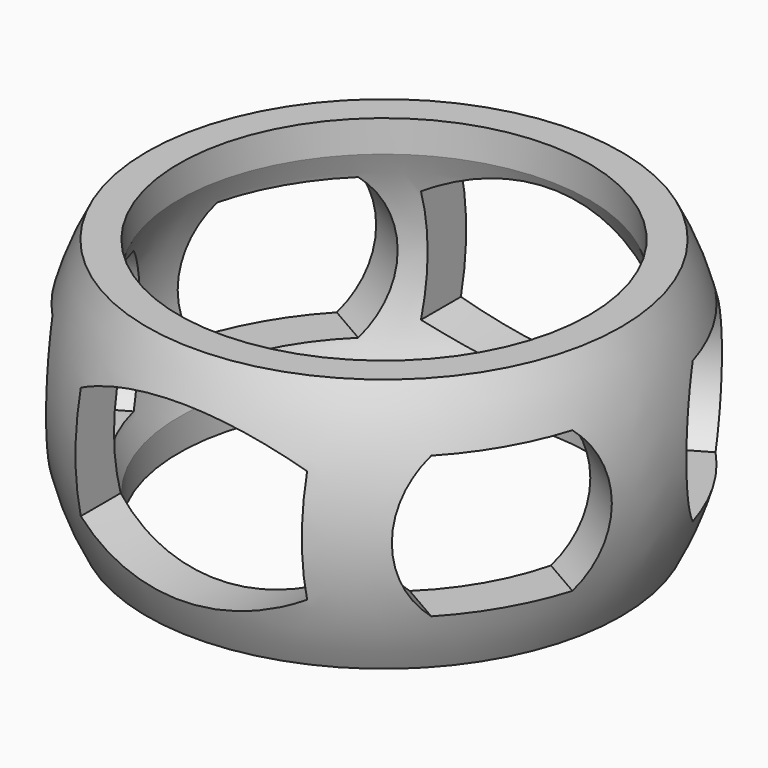
from build123d import *

# Parameters (mm, degrees)
F3_W      = 25.4
F3_H      = 12.7
F4_DEPTH  = 72.39
F7_DEPTH  = 53.086
F10_DEPTH = 47.244


# Not quite as in the source:
# - a feature names something its author has since deleted; it is built from what else it names


with BuildPart() as f1:
    # F0 (on Front) → F1 (revolve)
    with BuildSketch(Plane.XZ):
        with BuildLine():
            ThreePointArc((23.01875, 10.7376509739), (25.4, 0), (23.01875, -10.7376509739))
            Line((23.01875, -10.7376509739), (23.01875, -14.2875))
            Line((23.01875, -14.2875), (26.611533725, -14.2875))
            ThreePointArc((26.611533725, -14.2875), (30.20441, 0), (26.611533725, 14.2875))
            Line((26.611533725, 14.2875), (23.01875, 14.2875))
            Line((23.01875, 14.2875), (23.01875, 10.7376509739))
        make_face()
    revolve(axis=Axis((0, 0, -4.5421977431), (0, 0, -1)))

    # F3 (on offset) → F4 (cut)
    with BuildSketch(Plane.XZ.offset(30.20441)):
        with BuildLine():
            ThreePointArc((12.7, 6.35), (0, 9.7529547439), (-12.7, 6.35))
            Line((-12.7, 6.35), (12.7, 6.35))
        make_face()
        Rectangle(F3_W, F3_H)
        with BuildLine():
            Line((12.7, -6.35), (-12.7, -6.35))
            ThreePointArc((-12.7, -6.35), (0, -9.7529547439), (12.7, -6.35))
        make_face()
    extrude(amount=-F4_DEPTH, mode=Mode.SUBTRACT)

    # F6 (on line) → F7 (cut, symmetric)
    with BuildSketch(Plane(origin=(0, 0, 0), x_dir=(0.5, -0.8660254038, 0), z_dir=(-0.8660254038, -0.5, 0))):
        with BuildLine():
            ThreePointArc((6.6390036837, -7.9375), (10.34796, 0), (6.6390036837, 7.9375))
            Line((6.6390036837, 7.9375), (-6.6390036837, 7.9375))
            ThreePointArc((-6.6390036837, 7.9375), (-10.34796, 0), (-6.6390036837, -7.9375))
            Line((-6.6390036837, -7.9375), (6.6390036837, -7.9375))
        make_face()
    extrude(amount=F7_DEPTH, both=True, mode=Mode.SUBTRACT)

    # F9 (on line) → F10 (cut, symmetric)
    with BuildSketch(Plane(origin=(0, 0, 0), x_dir=(-0.5, -0.8660254038, 0), z_dir=(-0.8660254038, 0.5, 0))):
        with BuildLine():
            ThreePointArc((6.6390036837, -7.9375), (10.34796, 0), (6.6390036837, 7.9375))
            Line((6.6390036837, 7.9375), (-6.6390036837, 7.9375))
            ThreePointArc((-6.6390036837, 7.9375), (-10.34796, 0), (-6.6390036837, -7.9375))
            Line((-6.6390036837, -7.9375), (6.6390036837, -7.9375))
        make_face()
    extrude(amount=F10_DEPTH, both=True, mode=Mode.SUBTRACT)


solid = f1.part
